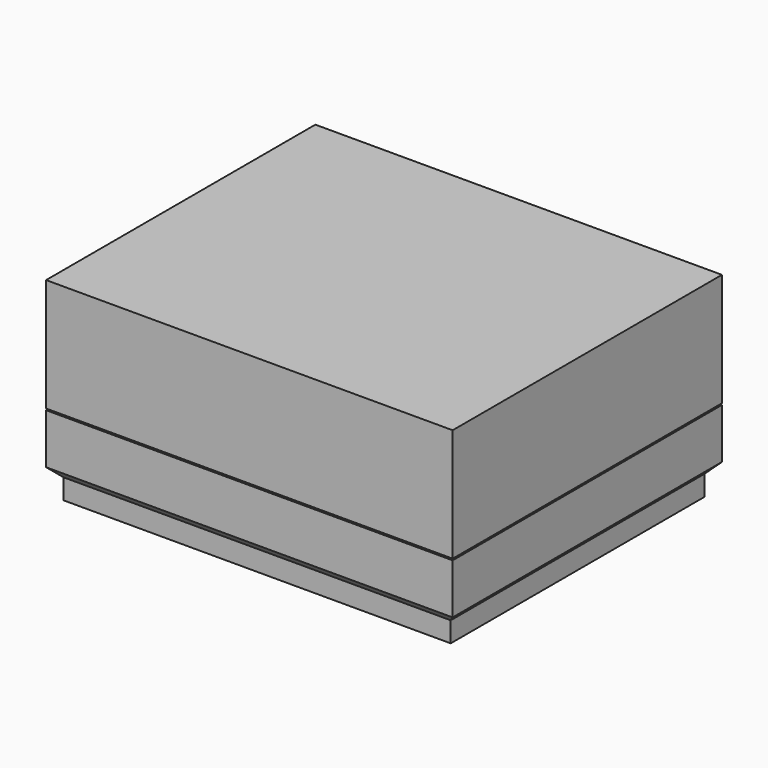
from build123d import *

# Parameters (mm, degrees)
F4_W          = 80.2
F4_H          = 66.4
F5_DEPTH      = 1
F6_W          = 80.2
F6_H          = 66.4
F6_W_2        = 73.2
F6_H_2        = 59.4
F7_DEPTH      = 18.1
F8_W          = 2
F8_H          = 18.1
F9_DEPTH      = 59.4
F12_W         = 80.2
F12_H         = 66.4
F12_W_2       = 76.4
F12_H_2       = 62.6
F13_DEPTH     = 3.3
F14_W         = 80.2
F14_H         = 66.4
F14_W_2       = 76.4
F14_H_2       = 62.6
F15_DEPTH     = 6
F16_T4_DEPTH  = 76.4
F16_T9_DEPTH  = 62.6
F16_T14_DEPTH = 76.4
F16_T19_DEPTH = 62.6
F16_T25_DEPTH = 81.5433659759
F16_T31_DEPTH = 67.7433659759
F16_T40_DEPTH = 81.5433659759
F16_T46_DEPTH = 67.7433659759
F16_T55_DEPTH = 81.5433659759
F16_T61_DEPTH = 67.7433659759
F16_T70_DEPTH = 67.7433659759
F16_T76_DEPTH = 81.5433659759
F17_W         = 80.2
F17_H         = 66.4
F17_W_2       = 77
F17_H_2       = 63.2
F18_DEPTH     = 3.2


# Not quite as in the source:
# - a fillet or chamfer that OpenCascade refuses, or shapes differently, is made with other operations: its cross-section is extruded or revolved along the edge and cut away or added
# - a feature names something its author has since deleted; it is built from what else it names


with BuildPart() as f5:
    # F4 (on Top) → F5 (new body)
    with BuildSketch(Plane.XY):
        Rectangle(F4_W, F4_H)
    extrude(amount=F5_DEPTH)

    # F6 (on face) → F7 (join)
    with BuildSketch(Plane.XY.offset(1)):
        Rectangle(F6_W, F6_H)
        Rectangle(F6_W_2, F6_H_2, mode=Mode.SUBTRACT)
    extrude(amount=F7_DEPTH)

    # F8 (on face) → F9 (join, through all)
    with BuildSketch(Plane.XZ.offset(-29.7)):
        with Locations((0, 10.05)):
            Rectangle(F8_W, F8_H)
    extrude(amount=F9_DEPTH)


with BuildPart() as f11_1:
    # F11: instance of F5
    add(f5.part.mirror(Plane.XY.offset(19.2)))

    # F17 (on face) → F18 (join)
    with BuildSketch(Plane(origin=(0, 0, 19.3), x_dir=(1, 0, 0), z_dir=(0, 0, -1))):
        Rectangle(F17_W, F17_H)
        Rectangle(F17_W_2, F17_H_2, mode=Mode.SUBTRACT)
    extrude(amount=F18_DEPTH)


with BuildPart() as f5_1:
    add(f5.part)

    # F12 (on face) → F13 (cut)
    with BuildSketch(Plane.XY.offset(19.1)):
        Rectangle(F12_W, F12_H)
        Rectangle(F12_W_2, F12_H_2, mode=Mode.SUBTRACT)
    extrude(amount=-F13_DEPTH, mode=Mode.SUBTRACT)

    # F14 (on face) → F15 (cut)
    with BuildSketch(Plane(origin=(0, 0, 0), x_dir=(1, 0, 0), z_dir=(0, 0, -1))):
        Rectangle(F14_W, F14_H)
        Rectangle(F14_W_2, F14_H_2, mode=Mode.SUBTRACT)
    extrude(amount=-F15_DEPTH, mode=Mode.SUBTRACT)

    # F16: chamfer of 2 on 4 edges, made by hand


with BuildPart() as f16_tool2:
    # F16_s3 → F16_t4 (new body)
    with BuildSketch(Plane.YZ.offset(-38.2)):
        Polygon((-33.3, 6), (-31.3, 4), (-31.3, 6), align=None)
    extrude(amount=F16_T4_DEPTH)

    split(bisect_by=Plane.XZ.offset(33.2), keep=Keep.BOTTOM)


with BuildPart() as f5_2:
    add(f5_1.part)

    # F16_t1: union F16_tool2
    add(f16_tool2.part)


with BuildPart() as f16_tool7:
    # F16_s8 → F16_t9 (new body)
    with BuildSketch(Plane.XZ.offset(-31.3)):
        Polygon((-40.2, 6), (-38.2, 4), (-38.2, 6), align=None)
    extrude(amount=F16_T9_DEPTH)

    split(bisect_by=Plane.YZ.offset(-40.1), keep=Keep.TOP)


with BuildPart() as f5_3:
    add(f5_2.part)

    # F16_t6: union F16_tool7
    add(f16_tool7.part)


with BuildPart() as f16_tool12:
    # F16_s13 → F16_t14 (new body)
    with BuildSketch(Plane.YZ.offset(38.2)):
        Polygon((33.3, 6), (31.3, 4), (31.3, 6), align=None)
    extrude(amount=-F16_T14_DEPTH)

    split(bisect_by=Plane.XZ.offset(-33.2), keep=Keep.TOP)


with BuildPart() as f5_4:
    add(f5_3.part)

    # F16_t11: union F16_tool12
    add(f16_tool12.part)


with BuildPart() as f16_tool17:
    # F16_s18 → F16_t19 (new body)
    with BuildSketch(Plane.XZ.offset(31.3)):
        Polygon((40.2, 6), (38.2, 4), (38.2, 6), align=None)
    extrude(amount=-F16_T19_DEPTH)

    split(bisect_by=Plane.YZ.offset(40.1), keep=Keep.BOTTOM)


with BuildPart() as f5_5:
    add(f5_4.part)

    # F16_t16: union F16_tool17
    add(f16_tool17.part)


with BuildPart() as f16_tool23:
    # F16_s24 → F16_t25 (new body)
    with BuildSketch(Plane.YZ.offset(-43.3433659759)):
        Polygon((-33.3, 6), (-31.3, 4), (-31.3, 6), align=None)
    extrude(amount=F16_T25_DEPTH)

    split(bisect_by=Plane.XZ.offset(33.2), keep=Keep.BOTTOM)

    split(bisect_by=Plane.YZ.offset(-40.1), keep=Keep.TOP)

    split(bisect_by=Plane.YZ.offset(-38.2), keep=Keep.BOTTOM)


with BuildPart() as f16_tool29:
    # F16_s30 → F16_t31 (new body)
    with BuildSketch(Plane.XZ.offset(-31.3)):
        Polygon((-40.2, 6), (-38.2, 4), (-38.2, 6), align=None)
    extrude(amount=F16_T31_DEPTH)

    split(bisect_by=Plane.XZ.offset(33.2), keep=Keep.BOTTOM)

    split(bisect_by=Plane.YZ.offset(-40.1), keep=Keep.TOP)

    split(bisect_by=Plane.XZ.offset(31.3), keep=Keep.TOP)


with BuildPart() as f16_tool23_1:
    add(f16_tool23.part)

    # F16_t35: intersect F16_tool29
    add(f16_tool29.part, mode=Mode.INTERSECT)


with BuildPart() as f5_6:
    add(f5_5.part)

    # F16_t21: union F16_tool23
    add(f16_tool23_1.part)


with BuildPart() as f16_tool38:
    # F16_s39 → F16_t40 (new body)
    with BuildSketch(Plane.YZ.offset(-38.2)):
        Polygon((-33.3, 6), (-31.3, 4), (-31.3, 6), align=None)
    extrude(amount=F16_T40_DEPTH)

    split(bisect_by=Plane.XZ.offset(33.2), keep=Keep.BOTTOM)

    split(bisect_by=Plane.YZ.offset(40.1), keep=Keep.BOTTOM)

    split(bisect_by=Plane.YZ.offset(38.2), keep=Keep.TOP)


with BuildPart() as f16_tool44:
    # F16_s45 → F16_t46 (new body)
    with BuildSketch(Plane.XZ.offset(36.4433659759)):
        Polygon((40.2, 6), (38.2, 4), (38.2, 6), align=None)
    extrude(amount=-F16_T46_DEPTH)

    split(bisect_by=Plane.XZ.offset(33.2), keep=Keep.BOTTOM)

    split(bisect_by=Plane.YZ.offset(40.1), keep=Keep.BOTTOM)

    split(bisect_by=Plane.XZ.offset(31.3), keep=Keep.TOP)


with BuildPart() as f16_tool38_1:
    add(f16_tool38.part)

    # F16_t50: intersect F16_tool44
    add(f16_tool44.part, mode=Mode.INTERSECT)


with BuildPart() as f5_7:
    add(f5_6.part)

    # F16_t36: union F16_tool38
    add(f16_tool38_1.part)


with BuildPart() as f16_tool53:
    # F16_s54 → F16_t55 (new body)
    with BuildSketch(Plane.YZ.offset(38.2)):
        Polygon((33.3, 6), (31.3, 4), (31.3, 6), align=None)
    extrude(amount=-F16_T55_DEPTH)

    split(bisect_by=Plane.YZ.offset(-40.1), keep=Keep.TOP)

    split(bisect_by=Plane.XZ.offset(-33.2), keep=Keep.TOP)

    split(bisect_by=Plane.YZ.offset(-38.2), keep=Keep.BOTTOM)


with BuildPart() as f16_tool59:
    # F16_s60 → F16_t61 (new body)
    with BuildSketch(Plane.XZ.offset(-36.4433659759)):
        Polygon((-40.2, 6), (-38.2, 4), (-38.2, 6), align=None)
    extrude(amount=F16_T61_DEPTH)

    split(bisect_by=Plane.YZ.offset(-40.1), keep=Keep.TOP)

    split(bisect_by=Plane.XZ.offset(-33.2), keep=Keep.TOP)

    split(bisect_by=Plane.XZ.offset(-31.3), keep=Keep.BOTTOM)


with BuildPart() as f16_tool53_1:
    add(f16_tool53.part)

    # F16_t65: intersect F16_tool59
    add(f16_tool59.part, mode=Mode.INTERSECT)


with BuildPart() as f5_8:
    add(f5_7.part)

    # F16_t51: union F16_tool53
    add(f16_tool53_1.part)


with BuildPart() as f16_tool68:
    # F16_s69 → F16_t70 (new body)
    with BuildSketch(Plane.XZ.offset(31.3)):
        Polygon((40.2, 6), (38.2, 4), (38.2, 6), align=None)
    extrude(amount=-F16_T70_DEPTH)

    split(bisect_by=Plane.YZ.offset(40.1), keep=Keep.BOTTOM)

    split(bisect_by=Plane.XZ.offset(-33.2), keep=Keep.TOP)

    split(bisect_by=Plane.XZ.offset(-31.3), keep=Keep.BOTTOM)


with BuildPart() as f16_tool74:
    # F16_s75 → F16_t76 (new body)
    with BuildSketch(Plane.YZ.offset(43.3433659759)):
        Polygon((33.3, 6), (31.3, 4), (31.3, 6), align=None)
    extrude(amount=-F16_T76_DEPTH)

    split(bisect_by=Plane.YZ.offset(40.1), keep=Keep.BOTTOM)

    split(bisect_by=Plane.XZ.offset(-33.2), keep=Keep.TOP)

    split(bisect_by=Plane.YZ.offset(38.2), keep=Keep.TOP)


with BuildPart() as f16_tool68_1:
    add(f16_tool68.part)

    # F16_t80: intersect F16_tool74
    add(f16_tool74.part, mode=Mode.INTERSECT)


with BuildPart() as f5_9:
    add(f5_8.part)

    # F16_t66: union F16_tool68
    add(f16_tool68_1.part)


solid = Compound([f11_1.part, f5_9.part])
